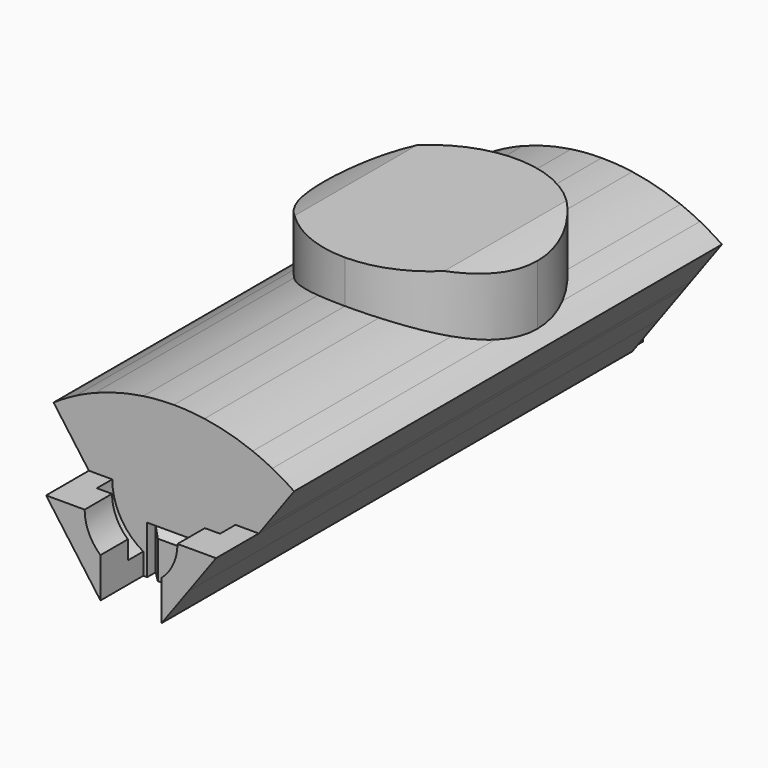
from build123d import *

# Parameters (mm, degrees)
F1_DEPTH     = 31.75
F2_DEPTH     = 3.175
F3_DEPTH     = 1.143
F4_DEPTH     = 32.8422
F7_DEPTH     = 5.08
F8_R         = 19.05
F8_R_2       = 15.875
F9_DEPTH     = 50.8
F11_SIZE     = 0.635
F12_T1_DEPTH = 10.9569141407


# Not quite as in the source:
# - a fillet or chamfer that OpenCascade refuses, or shapes differently, is made with other operations: its cross-section is extruded or revolved along the edge and cut away or added


with BuildPart() as f1:
    # F0 (on Front) → F1 (new body)
    with BuildSketch(Plane.XZ):
        with BuildLine():
            Line((-3.96875, 7.62), (-5.0456895848, 7.62))
            Line((-5.0456895848, 7.62), (-3.4113577324, 5.3705351863))
            Line((-3.4113577324, 5.3705351863), (-1.8162080478, 3.175))
            Line((-1.8162080478, 3.175), (-1.8162080478, 4.0912091463))
            ThreePointArc((-1.8162080478, 4.0912091463), (-3.3881449388, 5.5532512402), (-3.96875, 7.62))
        make_face()
        with BuildLine():
            Line((-5.2922131397, 7.9593105639), (-5.0456895848, 7.62))
            Line((-5.0456895848, 7.62), (-3.96875, 7.62))
            ThreePointArc((-3.96875, 7.62), (-3.3881449388, 9.6867487598), (-1.8162080478, 11.1487908537))
            Line((-1.8162080478, 11.1487908537), (-1.8162080478, 11.2776))
            Line((-1.8162080478, 11.2776), (-4.4524904002, 11.2776))
            ThreePointArc((-4.4524904002, 11.2776), (-4.386898372, 9.4956069696), (-5.2922131397, 7.9593105639))
        make_face()
        with BuildLine():
            Line((-1.8162080478, 4.0912091463), (-1.8162080478, 3.175))
            Line((-1.8162080478, 3.175), (-1.5875, 3.175))
            Line((-1.5875, 3.175), (-1.5875, 3.9825805421))
            ThreePointArc((-1.5875, 3.9825805421), (-1.7027205179, 4.0350705167), (-1.8162080478, 4.0912091463))
        make_face()
        with BuildLine():
            Line((3.96875, 7.62), (5.0456895848, 7.62))
            Line((5.0456895848, 7.62), (5.2922131397, 7.9593105639))
            ThreePointArc((5.2922131397, 7.9593105639), (4.386898372, 9.4956069696), (4.4524904002, 11.2776))
            Line((4.4524904002, 11.2776), (1.8162080478, 11.2776))
            Line((1.8162080478, 11.2776), (1.8162080478, 11.1487908537))
            ThreePointArc((1.8162080478, 11.1487908537), (3.3881449388, 9.6867487598), (3.96875, 7.62))
        make_face()
        with BuildLine():
            Line((3.4113577324, 5.3705351863), (5.0456895848, 7.62))
            Line((5.0456895848, 7.62), (3.96875, 7.62))
            ThreePointArc((3.96875, 7.62), (3.3881449388, 5.5532512402), (1.8162080478, 4.0912091463))
            Line((1.8162080478, 4.0912091463), (1.8162080478, 3.175))
            Line((1.8162080478, 3.175), (3.4113577324, 5.3705351863))
        make_face()
        with BuildLine():
            Line((1.5875, 3.175), (1.8162080478, 3.175))
            Line((1.8162080478, 3.175), (1.8162080478, 4.0912091463))
            ThreePointArc((1.8162080478, 4.0912091463), (1.7027205179, 4.0350705167), (1.5875, 3.9825805421))
            Line((1.5875, 3.9825805421), (1.5875, 3.175))
        make_face()
        with BuildLine():
            Line((-7.1401482368, 10.5027750217), (-5.2922131397, 7.9593105639))
            ThreePointArc((-5.2922131397, 7.9593105639), (-4.386898372, 9.4956069696), (-4.4524904002, 11.2776))
            Line((-4.4524904002, 11.2776), (-5.8400118356, 11.2776))
            ThreePointArc((-5.8400118356, 11.2776), (-6.5016326652, 10.9095725254), (-7.1401482368, 10.5027750217))
        make_face()
        with BuildLine():
            Line((-3.6576, 7.62), (-3.96875, 7.62))
            ThreePointArc((-3.96875, 7.62), (-3.3881449388, 5.5532512402), (-1.8162080478, 4.0912091463))
            Line((-1.8162080478, 4.0912091463), (-1.8162080478, 4.4451888108))
            ThreePointArc((-1.8162080478, 4.4451888108), (-3.1639374453, 5.7849148243), (-3.6576, 7.62))
        make_face()
        with BuildLine():
            ThreePointArc((-1.8162080478, 11.1487908537), (-3.3881449388, 9.6867487598), (-3.96875, 7.62))
            Line((-3.96875, 7.62), (-3.6576, 7.62))
            ThreePointArc((-3.6576, 7.62), (-3.1639374453, 9.4550851757), (-1.8162080478, 10.7948111892))
            Line((-1.8162080478, 10.7948111892), (-1.8162080478, 11.1487908537))
        make_face()
        with BuildLine():
            Line((-1.8162080478, 4.4451888108), (-1.8162080478, 4.0912091463))
            ThreePointArc((-1.8162080478, 4.0912091463), (-1.7027205179, 4.0350705167), (-1.5875, 3.9825805421))
            Line((-1.5875, 3.9825805421), (-1.5875, 4.3248700314))
            ThreePointArc((-1.5875, 4.3248700314), (-1.7029169889, 4.3830088834), (-1.8162080478, 4.4451888108))
        make_face()
        with BuildLine():
            ThreePointArc((4.4524904002, 11.2776), (4.386898372, 9.4956069696), (5.2922131397, 7.9593105639))
            Line((5.2922131397, 7.9593105639), (7.1401482368, 10.5027750217))
            ThreePointArc((7.1401482368, 10.5027750217), (6.5016326652, 10.9095725254), (5.8400118356, 11.2776))
            Line((5.8400118356, 11.2776), (4.4524904002, 11.2776))
        make_face()
        with BuildLine():
            Line((3.6576, 7.62), (3.96875, 7.62))
            ThreePointArc((3.96875, 7.62), (3.3881449388, 9.6867487598), (1.8162080478, 11.1487908537))
            Line((1.8162080478, 11.1487908537), (1.8162080478, 10.7948111892))
            ThreePointArc((1.8162080478, 10.7948111892), (3.1639374453, 9.4550851757), (3.6576, 7.62))
        make_face()
        with BuildLine():
            ThreePointArc((1.8162080478, 4.0912091463), (3.3881449388, 5.5532512402), (3.96875, 7.62))
            Line((3.96875, 7.62), (3.6576, 7.62))
            ThreePointArc((3.6576, 7.62), (3.1639374453, 5.7849148243), (1.8162080478, 4.4451888108))
            Line((1.8162080478, 4.4451888108), (1.8162080478, 4.0912091463))
        make_face()
        with BuildLine():
            ThreePointArc((1.5875, 3.9825805421), (1.7027205179, 4.0350705167), (1.8162080478, 4.0912091463))
            Line((1.8162080478, 4.0912091463), (1.8162080478, 4.4451888108))
            ThreePointArc((1.8162080478, 4.4451888108), (1.7029169889, 4.3830088834), (1.5875, 4.3248700314))
            Line((1.5875, 4.3248700314), (1.5875, 3.9825805421))
        make_face()
        with BuildLine():
            ThreePointArc((-4.6831128955, 11.8050181537), (-4.5558242029, 11.5465464169), (-4.4524904002, 11.2776))
            Line((-4.4524904002, 11.2776), (-1.8162080478, 11.2776))
            Line((-1.8162080478, 11.2776), (-1.8162080478, 12.5694625313))
            ThreePointArc((-1.8162080478, 12.5694625313), (-3.2720615799, 12.2712514854), (-4.6831128955, 11.8050181537))
        make_face()
        with BuildLine():
            Line((-5.8400118356, 11.2776), (-4.4524904002, 11.2776))
            ThreePointArc((-4.4524904002, 11.2776), (-4.5558242029, 11.5465464169), (-4.6831128955, 11.8050181537))
            ThreePointArc((-4.6831128955, 11.8050181537), (-5.2681667593, 11.5557959049), (-5.8400118356, 11.2776))
        make_face()
        with BuildLine():
            Line((-1.8162080478, 11.2776), (-1.8162080478, 11.1487908537))
            ThreePointArc((-1.8162080478, 11.1487908537), (-1.6795566201, 11.2158401136), (-1.5404346148, 11.2776))
            Line((-1.5404346148, 11.2776), (-1.8162080478, 11.2776))
        make_face()
        with BuildLine():
            ThreePointArc((-1.5404346148, 11.2776), (-1.6795566201, 11.2158401136), (-1.8162080478, 11.1487908537))
            Line((-1.8162080478, 11.1487908537), (-1.8162080478, 10.7948111892))
            ThreePointArc((-1.8162080478, 10.7948111892), (-0.939640451, 11.1548427946), (0, 11.2776))
            Line((0, 11.2776), (-1.5404346148, 11.2776))
        make_face()
        with BuildLine():
            Line((-2.7559, 7.62), (-3.6576, 7.62))
            ThreePointArc((-3.6576, 7.62), (-3.1639374453, 5.7849148243), (-1.8162080478, 4.4451888108))
            Line((-1.8162080478, 4.4451888108), (-1.8162080478, 5.5472305635))
            ThreePointArc((-1.8162080478, 5.5472305635), (-2.510007228, 6.4820858884), (-2.7559, 7.62))
        make_face()
        with BuildLine():
            ThreePointArc((-1.8162080478, 10.7948111892), (-3.1639374453, 9.4550851757), (-3.6576, 7.62))
            Line((-3.6576, 7.62), (-2.7559, 7.62))
            ThreePointArc((-2.7559, 7.62), (-2.510007228, 8.7579141116), (-1.8162080478, 9.6927694365))
            Line((-1.8162080478, 9.6927694365), (-1.8162080478, 10.7948111892))
        make_face()
        with BuildLine():
            Line((-1.8162080478, 5.5472305635), (-1.8162080478, 4.4451888108))
            ThreePointArc((-1.8162080478, 4.4451888108), (-1.7029169889, 4.3830088834), (-1.5875, 4.3248700314))
            Line((-1.5875, 4.3248700314), (-1.5875, 5.3672619859))
            ThreePointArc((-1.5875, 5.3672619859), (-1.7042312903, 5.454225192), (-1.8162080478, 5.5472305635))
        make_face()
        with BuildLine():
            ThreePointArc((4.6831128955, 11.8050181537), (4.5558242029, 11.5465464169), (4.4524904002, 11.2776))
            Line((4.4524904002, 11.2776), (5.8400118356, 11.2776))
            ThreePointArc((5.8400118356, 11.2776), (5.2681667593, 11.5557959049), (4.6831128955, 11.8050181537))
        make_face()
        with BuildLine():
            Line((1.8162080478, 11.2776), (4.4524904002, 11.2776))
            ThreePointArc((4.4524904002, 11.2776), (4.5558242029, 11.5465464169), (4.6831128955, 11.8050181537))
            ThreePointArc((4.6831128955, 11.8050181537), (3.2720615799, 12.2712514854), (1.8162080478, 12.5694625313))
            Line((1.8162080478, 12.5694625313), (1.8162080478, 11.2776))
        make_face()
        with BuildLine():
            Line((1.8162080478, 10.7948111892), (1.8162080478, 11.1487908537))
            ThreePointArc((1.8162080478, 11.1487908537), (1.6795566201, 11.2158401136), (1.5404346148, 11.2776))
            Line((1.5404346148, 11.2776), (0, 11.2776))
            ThreePointArc((0, 11.2776), (0.939640451, 11.1548427946), (1.8162080478, 10.7948111892))
        make_face()
        with BuildLine():
            ThreePointArc((1.5404346148, 11.2776), (1.6795566201, 11.2158401136), (1.8162080478, 11.1487908537))
            Line((1.8162080478, 11.1487908537), (1.8162080478, 11.2776))
            Line((1.8162080478, 11.2776), (1.5404346148, 11.2776))
        make_face()
        with BuildLine():
            Line((2.7559, 7.62), (3.6576, 7.62))
            ThreePointArc((3.6576, 7.62), (3.1639374453, 9.4550851757), (1.8162080478, 10.7948111892))
            Line((1.8162080478, 10.7948111892), (1.8162080478, 9.6927694365))
            ThreePointArc((1.8162080478, 9.6927694365), (2.510007228, 8.7579141116), (2.7559, 7.62))
        make_face()
        with BuildLine():
            ThreePointArc((1.8162080478, 4.4451888108), (3.1639374453, 5.7849148243), (3.6576, 7.62))
            Line((3.6576, 7.62), (2.7559, 7.62))
            ThreePointArc((2.7559, 7.62), (2.510007228, 6.4820858884), (1.8162080478, 5.5472305635))
            Line((1.8162080478, 5.5472305635), (1.8162080478, 4.4451888108))
        make_face()
        with BuildLine():
            ThreePointArc((1.5875, 4.3248700314), (1.7029169889, 4.3830088834), (1.8162080478, 4.4451888108))
            Line((1.8162080478, 4.4451888108), (1.8162080478, 5.5472305635))
            ThreePointArc((1.8162080478, 5.5472305635), (1.7042312903, 5.454225192), (1.5875, 5.3672619859))
            Line((1.5875, 5.3672619859), (1.5875, 4.3248700314))
        make_face()
        with BuildLine():
            Line((-1.8162080478, 12.5694625313), (-1.8162080478, 11.2776))
            Line((-1.8162080478, 11.2776), (-1.5404346148, 11.2776))
            ThreePointArc((-1.5404346148, 11.2776), (-0.7857724106, 11.5101848647), (0, 11.58875))
            Line((0, 11.58875), (0, 12.7))
            ThreePointArc((0, 12.7), (-0.910446553, 12.6673235955), (-1.8162080478, 12.5694625313))
        make_face()
        with BuildLine():
            ThreePointArc((0, 11.58875), (-0.7857724106, 11.5101848647), (-1.5404346148, 11.2776))
            Line((-1.5404346148, 11.2776), (0, 11.2776))
            Line((0, 11.2776), (0, 11.58875))
        make_face()
        with BuildLine():
            ThreePointArc((0, 11.2776), (-0.939640451, 11.1548427946), (-1.8162080478, 10.7948111892))
            Line((-1.8162080478, 10.7948111892), (-1.8162080478, 9.6927694365))
            ThreePointArc((-1.8162080478, 9.6927694365), (-0.970216347, 10.1994699165), (0, 10.3759))
            Line((0, 10.3759), (0, 11.2776))
        make_face()
        with BuildLine():
            Line((-1.8162080478, 7.62), (-2.7559, 7.62))
            ThreePointArc((-2.7559, 7.62), (-2.510007228, 6.4820858884), (-1.8162080478, 5.5472305635))
            Line((-1.8162080478, 5.5472305635), (-1.8162080478, 6.0325))
            Line((-1.8162080478, 6.0325), (-1.8162080478, 7.62))
        make_face()
        with BuildLine():
            ThreePointArc((-1.8162080478, 9.6927694365), (-2.510007228, 8.7579141116), (-2.7559, 7.62))
            Line((-2.7559, 7.62), (-1.8162080478, 7.62))
            Line((-1.8162080478, 7.62), (-1.8162080478, 9.525))
            Line((-1.8162080478, 9.525), (-1.8162080478, 9.6927694365))
        make_face()
        with BuildLine():
            Line((-1.8162080478, 6.0325), (-1.8162080478, 5.5472305635))
            ThreePointArc((-1.8162080478, 5.5472305635), (-1.7042312903, 5.454225192), (-1.5875, 5.3672619859))
            Line((-1.5875, 5.3672619859), (-1.5875, 6.0325))
            Line((-1.5875, 6.0325), (-1.8162080478, 6.0325))
        make_face()
        with BuildLine():
            Line((1.5404346148, 11.2776), (1.8162080478, 11.2776))
            Line((1.8162080478, 11.2776), (1.8162080478, 12.5694625313))
            ThreePointArc((1.8162080478, 12.5694625313), (0.910446553, 12.6673235955), (0, 12.7))
            Line((0, 12.7), (0, 11.58875))
            ThreePointArc((0, 11.58875), (0.7857724106, 11.5101848647), (1.5404346148, 11.2776))
        make_face()
        with BuildLine():
            Line((0, 11.2776), (1.5404346148, 11.2776))
            ThreePointArc((1.5404346148, 11.2776), (0.7857724106, 11.5101848647), (0, 11.58875))
            Line((0, 11.58875), (0, 11.2776))
        make_face()
        with BuildLine():
            Line((1.8162080478, 9.6927694365), (1.8162080478, 10.7948111892))
            ThreePointArc((1.8162080478, 10.7948111892), (0.939640451, 11.1548427946), (0, 11.2776))
            Line((0, 11.2776), (0, 10.3759))
            ThreePointArc((0, 10.3759), (0.970216347, 10.1994699165), (1.8162080478, 9.6927694365))
        make_face()
        with BuildLine():
            Line((1.8162080478, 7.62), (2.7559, 7.62))
            ThreePointArc((2.7559, 7.62), (2.510007228, 8.7579141116), (1.8162080478, 9.6927694365))
            Line((1.8162080478, 9.6927694365), (1.8162080478, 9.525))
            Line((1.8162080478, 9.525), (1.8162080478, 7.62))
        make_face()
        with BuildLine():
            ThreePointArc((1.8162080478, 5.5472305635), (2.510007228, 6.4820858884), (2.7559, 7.62))
            Line((2.7559, 7.62), (1.8162080478, 7.62))
            Line((1.8162080478, 7.62), (1.8162080478, 6.0325))
            Line((1.8162080478, 6.0325), (1.8162080478, 5.5472305635))
        make_face()
        with BuildLine():
            ThreePointArc((1.5875, 5.3672619859), (1.7042312903, 5.454225192), (1.8162080478, 5.5472305635))
            Line((1.8162080478, 5.5472305635), (1.8162080478, 6.0325))
            Line((1.8162080478, 6.0325), (1.5875, 6.0325))
            Line((1.5875, 6.0325), (1.5875, 5.3672619859))
        make_face()
        Polygon((-1.5875, 6.0325), (0, 6.0325), (1.5875, 6.0325), (1.8162080478, 6.0325), (1.8162080478, 7.62), (0, 7.62), (-1.8162080478, 7.62), (-1.8162080478, 6.0325), align=None)
        with BuildLine():
            ThreePointArc((0, 10.3759), (-0.970216347, 10.1994699165), (-1.8162080478, 9.6927694365))
            Line((-1.8162080478, 9.6927694365), (-1.8162080478, 9.525))
            Line((-1.8162080478, 9.525), (0, 9.525))
            Line((0, 9.525), (0, 10.3759))
        make_face()
        Polygon((-1.8162080478, 9.525), (-1.8162080478, 7.62), (0, 7.62), (1.8162080478, 7.62), (1.8162080478, 9.525), (0, 9.525), align=None)
        with BuildLine():
            Line((1.8162080478, 9.525), (1.8162080478, 9.6927694365))
            ThreePointArc((1.8162080478, 9.6927694365), (0.970216347, 10.1994699165), (0, 10.3759))
            Line((0, 10.3759), (0, 9.525))
            Line((0, 9.525), (1.8162080478, 9.525))
        make_face()
    extrude(amount=-F1_DEPTH)

    # F0 (on Front) → F2 (join)
    with BuildSketch(Plane.XZ):
        with BuildLine():
            Line((-3.96875, 7.62), (-5.0456895848, 7.62))
            Line((-5.0456895848, 7.62), (-3.4113577324, 5.3705351863))
            Line((-3.4113577324, 5.3705351863), (-1.8162080478, 3.175))
            Line((-1.8162080478, 3.175), (-1.8162080478, 4.0912091463))
            ThreePointArc((-1.8162080478, 4.0912091463), (-3.3881449388, 5.5532512402), (-3.96875, 7.62))
        make_face()
        with BuildLine():
            Line((3.4113577324, 5.3705351863), (5.0456895848, 7.62))
            Line((5.0456895848, 7.62), (3.96875, 7.62))
            ThreePointArc((3.96875, 7.62), (3.3881449388, 5.5532512402), (1.8162080478, 4.0912091463))
            Line((1.8162080478, 4.0912091463), (1.8162080478, 3.175))
            Line((1.8162080478, 3.175), (3.4113577324, 5.3705351863))
        make_face()
        with BuildLine():
            Line((-3.6576, 7.62), (-3.96875, 7.62))
            ThreePointArc((-3.96875, 7.62), (-3.3881449388, 5.5532512402), (-1.8162080478, 4.0912091463))
            Line((-1.8162080478, 4.0912091463), (-1.8162080478, 4.4451888108))
            ThreePointArc((-1.8162080478, 4.4451888108), (-3.1639374453, 5.7849148243), (-3.6576, 7.62))
        make_face()
        with BuildLine():
            ThreePointArc((1.8162080478, 4.0912091463), (3.3881449388, 5.5532512402), (3.96875, 7.62))
            Line((3.96875, 7.62), (3.6576, 7.62))
            ThreePointArc((3.6576, 7.62), (3.1639374453, 5.7849148243), (1.8162080478, 4.4451888108))
            Line((1.8162080478, 4.4451888108), (1.8162080478, 4.0912091463))
        make_face()
        with BuildLine():
            Line((-2.7559, 7.62), (-3.6576, 7.62))
            ThreePointArc((-3.6576, 7.62), (-3.1639374453, 5.7849148243), (-1.8162080478, 4.4451888108))
            Line((-1.8162080478, 4.4451888108), (-1.8162080478, 5.5472305635))
            ThreePointArc((-1.8162080478, 5.5472305635), (-2.510007228, 6.4820858884), (-2.7559, 7.62))
        make_face()
        with BuildLine():
            ThreePointArc((1.8162080478, 4.4451888108), (3.1639374453, 5.7849148243), (3.6576, 7.62))
            Line((3.6576, 7.62), (2.7559, 7.62))
            ThreePointArc((2.7559, 7.62), (2.510007228, 6.4820858884), (1.8162080478, 5.5472305635))
            Line((1.8162080478, 5.5472305635), (1.8162080478, 4.4451888108))
        make_face()
    extrude(amount=F2_DEPTH)

    # F0 (on Front) → F3 (cut)
    with BuildSketch(Plane.XZ):
        with BuildLine():
            Line((-2.7559, 7.62), (-3.6576, 7.62))
            ThreePointArc((-3.6576, 7.62), (-3.1639374453, 5.7849148243), (-1.8162080478, 4.4451888108))
            Line((-1.8162080478, 4.4451888108), (-1.8162080478, 5.5472305635))
            ThreePointArc((-1.8162080478, 5.5472305635), (-2.510007228, 6.4820858884), (-2.7559, 7.62))
        make_face()
        with BuildLine():
            ThreePointArc((1.8162080478, 4.4451888108), (3.1639374453, 5.7849148243), (3.6576, 7.62))
            Line((3.6576, 7.62), (2.7559, 7.62))
            ThreePointArc((2.7559, 7.62), (2.510007228, 6.4820858884), (1.8162080478, 5.5472305635))
            Line((1.8162080478, 5.5472305635), (1.8162080478, 4.4451888108))
        make_face()
        with BuildLine():
            Line((1.8162080478, 9.6927694365), (1.8162080478, 10.7948111892))
            ThreePointArc((1.8162080478, 10.7948111892), (0.939640451, 11.1548427946), (0, 11.2776))
            Line((0, 11.2776), (0, 10.3759))
            ThreePointArc((0, 10.3759), (0.970216347, 10.1994699165), (1.8162080478, 9.6927694365))
        make_face()
    extrude(amount=F3_DEPTH, mode=Mode.SUBTRACT)

    # F6 (on offset) → F7 (join)
    with BuildSketch(Plane.XY.offset(10.16)):
        with BuildLine():
            ThreePointArc((0, 12.7), (4.4901280605, 14.5598719395), (6.35, 19.05))
            ThreePointArc((6.35, 19.05), (-4.4901280605, 23.5401280605), (0, 12.7))
        make_face()
    extrude(amount=F7_DEPTH)

    # F8 (on Front) → F9 (cut)
    with BuildSketch(Plane.XZ):
        Circle(F8_R)
        Circle(F8_R_2, mode=Mode.SUBTRACT)
    extrude(amount=-F9_DEPTH, mode=Mode.SUBTRACT)


with BuildPart() as f4:
    # F0 (on Front) → F4 (new body)
    with BuildSketch(Plane.XZ):
        with BuildLine():
            ThreePointArc((-1.5875, 5.3672619859), (-0.8326656343, 4.9929003157), (0, 4.8641))
            Line((0, 4.8641), (0, 6.0325))
            Line((0, 6.0325), (-1.5875, 6.0325))
            Line((-1.5875, 6.0325), (-1.5875, 5.3672619859))
        make_face()
        with BuildLine():
            Line((0, 6.0325), (0, 4.8641))
            ThreePointArc((0, 4.8641), (0.8326656343, 4.9929003157), (1.5875, 5.3672619859))
            Line((1.5875, 5.3672619859), (1.5875, 6.0325))
            Line((1.5875, 6.0325), (0, 6.0325))
        make_face()
        with BuildLine():
            Line((0, 4.8641), (0, 3.9624))
            ThreePointArc((0, 3.9624), (0.8141776179, 4.0541687412), (1.5875, 4.3248700314))
            Line((1.5875, 4.3248700314), (1.5875, 5.3672619859))
            ThreePointArc((1.5875, 5.3672619859), (0.8326656343, 4.9929003157), (0, 4.8641))
        make_face()
        with BuildLine():
            ThreePointArc((-1.5875, 4.3248700314), (-0.8141776179, 4.0541687412), (0, 3.9624))
            Line((0, 3.9624), (0, 4.8641))
            ThreePointArc((0, 4.8641), (-0.8326656343, 4.9929003157), (-1.5875, 5.3672619859))
            Line((-1.5875, 5.3672619859), (-1.5875, 4.3248700314))
        make_face()
        with BuildLine():
            ThreePointArc((-1.5875, 3.9825805421), (-0.8108538984, 3.7349655706), (0, 3.65125))
            Line((0, 3.65125), (0, 3.9624))
            ThreePointArc((0, 3.9624), (-0.8141776179, 4.0541687412), (-1.5875, 4.3248700314))
            Line((-1.5875, 4.3248700314), (-1.5875, 3.9825805421))
        make_face()
        with BuildLine():
            Line((0, 3.9624), (0, 3.65125))
            ThreePointArc((0, 3.65125), (0.8108538984, 3.7349655706), (1.5875, 3.9825805421))
            Line((1.5875, 3.9825805421), (1.5875, 4.3248700314))
            ThreePointArc((1.5875, 4.3248700314), (0.8141776179, 4.0541687412), (0, 3.9624))
        make_face()
        with BuildLine():
            Line((0, 3.65125), (0, 3.175))
            Line((0, 3.175), (0.79375, 3.175))
            Line((0.79375, 3.175), (1.5875, 3.175))
            Line((1.5875, 3.175), (1.5875, 3.9825805421))
            ThreePointArc((1.5875, 3.9825805421), (0.8108538984, 3.7349655706), (0, 3.65125))
        make_face()
        with BuildLine():
            Line((-0.79375, 3.175), (0, 3.175))
            Line((0, 3.175), (0, 3.65125))
            ThreePointArc((0, 3.65125), (-0.8108538984, 3.7349655706), (-1.5875, 3.9825805421))
            Line((-1.5875, 3.9825805421), (-1.5875, 3.175))
            Line((-1.5875, 3.175), (-0.79375, 3.175))
        make_face()
    extrude(amount=-F4_DEPTH)

    # F11
    f11_edges = [f4.edges().sort_by_distance(p)[0] for p in [
        (-1.5875, 0, 4.60375),
        (1.5875, 0, 4.60375),
    ]]
    chamfer(f11_edges, length=F11_SIZE)

    # F12: chamfer of 0.635 x 1.7446481614 on 1 edges, made by hand

    # F12_s2 → F12_t1 (cut)
    with BuildSketch(Plane.YZ.offset(-5.4784570703)):
        Polygon((1.7446481614, 6.0325), (0, 5.3975), (0, 6.0325), align=None)
    extrude(amount=F12_T1_DEPTH, mode=Mode.SUBTRACT)


solid = Compound([f1.part, f4.part])
